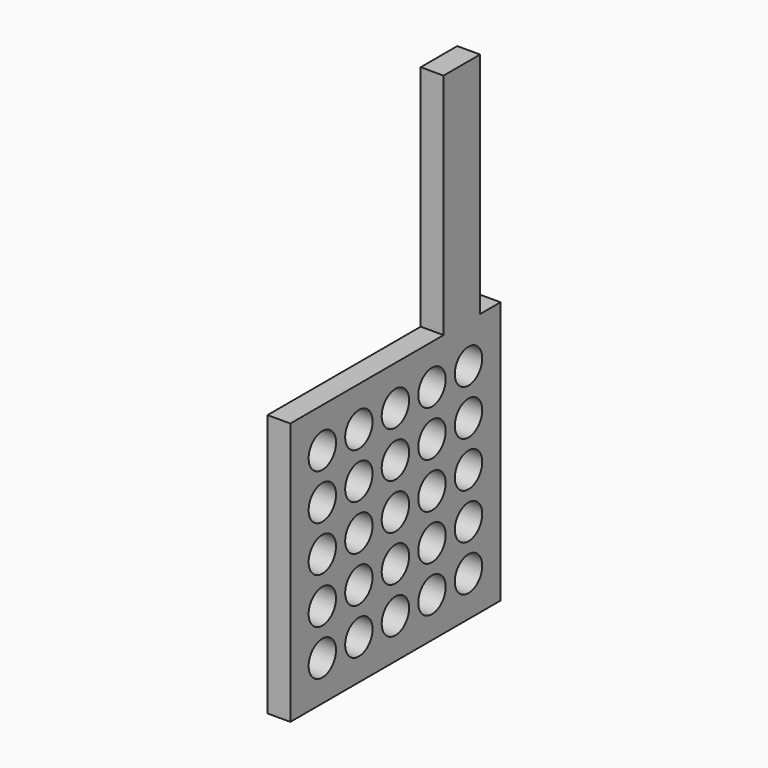
from build123d import *

# Parameters (mm, degrees)
F0_R     = 0.75
F1_DEPTH = 1


# Not quite as in the source:
# - a feature names something its author has since deleted; it is built from what else it names


with BuildPart() as f1:
    # F0 (on Right) → F1 (new body)
    with BuildSketch(Plane.YZ):
        Polygon((8.384144865, 0), (0, 0), (0, -11.5), (11.5, -11.5), (11.5, 0), (10.384144865, 0), (10.384144865, 10), (8.384144865, 10), align=None)
        with Locations((1.75, -9.75)):
            Circle(F0_R, mode=Mode.SUBTRACT)
        with Locations((1.75, -7.75)):
            Circle(F0_R, mode=Mode.SUBTRACT)
        with Locations((3.75, -9.75)):
            Circle(F0_R, mode=Mode.SUBTRACT)
        with Locations((3.75, -7.75)):
            Circle(F0_R, mode=Mode.SUBTRACT)
        with Locations((1.75, -5.75)):
            Circle(F0_R, mode=Mode.SUBTRACT)
        with Locations((1.75, -3.75)):
            Circle(F0_R, mode=Mode.SUBTRACT)
        with Locations((1.75, -1.75)):
            Circle(F0_R, mode=Mode.SUBTRACT)
        with Locations((3.75, -5.75)):
            Circle(F0_R, mode=Mode.SUBTRACT)
        with Locations((3.75, -3.75)):
            Circle(F0_R, mode=Mode.SUBTRACT)
        with Locations((3.75, -1.75)):
            Circle(F0_R, mode=Mode.SUBTRACT)
        with Locations((5.75, -9.75)):
            Circle(F0_R, mode=Mode.SUBTRACT)
        with Locations((7.75, -9.75)):
            Circle(F0_R, mode=Mode.SUBTRACT)
        with Locations((5.75, -7.75)):
            Circle(F0_R, mode=Mode.SUBTRACT)
        with Locations((7.75, -7.75)):
            Circle(F0_R, mode=Mode.SUBTRACT)
        with Locations((9.75, -9.75)):
            Circle(F0_R, mode=Mode.SUBTRACT)
        with Locations((9.75, -7.75)):
            Circle(F0_R, mode=Mode.SUBTRACT)
        with Locations((5.75, -5.75)):
            Circle(F0_R, mode=Mode.SUBTRACT)
        with Locations((5.75, -3.75)):
            Circle(F0_R, mode=Mode.SUBTRACT)
        with Locations((7.75, -5.75)):
            Circle(F0_R, mode=Mode.SUBTRACT)
        with Locations((7.75, -3.75)):
            Circle(F0_R, mode=Mode.SUBTRACT)
        with Locations((5.75, -1.75)):
            Circle(F0_R, mode=Mode.SUBTRACT)
        with Locations((7.75, -1.75)):
            Circle(F0_R, mode=Mode.SUBTRACT)
        with Locations((9.75, -5.75)):
            Circle(F0_R, mode=Mode.SUBTRACT)
        with Locations((9.75, -3.75)):
            Circle(F0_R, mode=Mode.SUBTRACT)
        with Locations((9.75, -1.75)):
            Circle(F0_R, mode=Mode.SUBTRACT)
    extrude(amount=F1_DEPTH)


solid = f1.part
